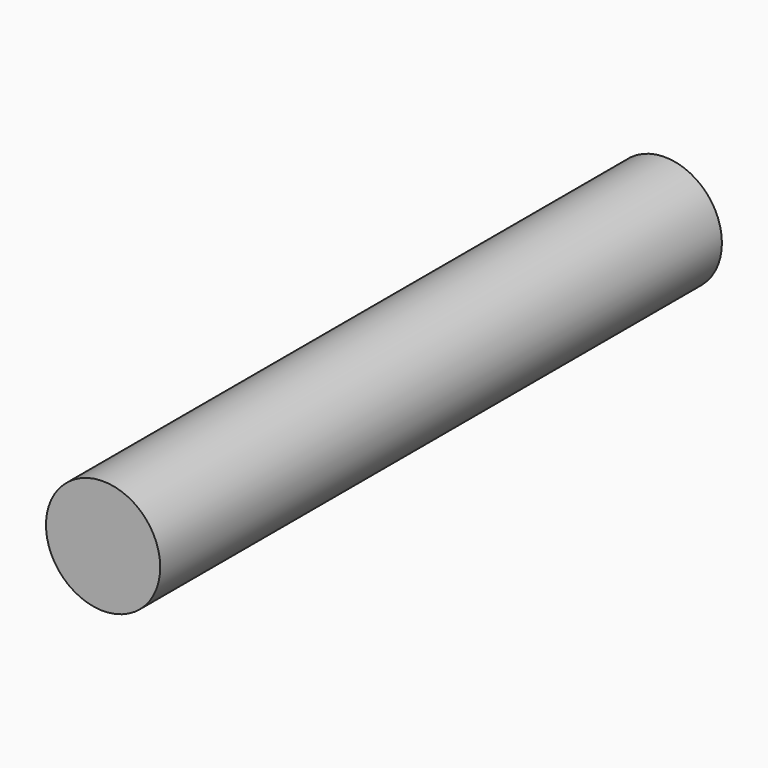
from build123d import *

# Parameters (mm, degrees)
F0_R     = 12.7
F1_DEPTH = 156.10424


# Not quite as in the source:
# - a feature of the source that left no trace in its solid (it failed there, or was rolled back) is left out
# - the program builds the solid bodies; features that only make, move or delete a surface that nothing else refers to are left out


with BuildPart() as f1:
    # F0 (on Front) → F1 (new body)
    with BuildSketch(Plane.XZ):
        Circle(F0_R)
    extrude(amount=F1_DEPTH)


solid = f1.part
